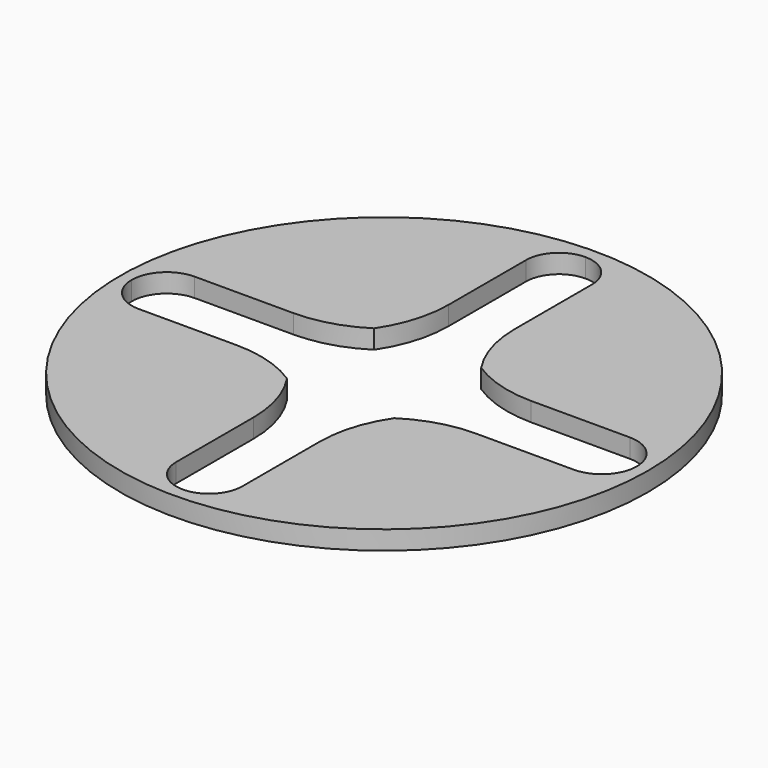
from build123d import *

# Parameters (mm, degrees)
F0_R        = 44.45
F0_R_2      = 12.7
F1_DEPTH    = 3.175
F3_DEPTH    = 25.4
F4_T1_DEPTH = 48.6343800889
F4_T3_DEPTH = 47.4571451006
F4_T5_DEPTH = 47.1924378771


# Not quite as in the source:
# - a fillet or chamfer that OpenCascade refuses, or shapes differently, is made with other operations: its cross-section is extruded or revolved along the edge and cut away or added


with BuildPart() as f1:
    # F0 (on Top) → F1 (new body)
    with BuildSketch(Plane.XY):
        Circle(F0_R)
        Circle(F0_R_2, mode=Mode.SUBTRACT)
    extrude(amount=F1_DEPTH)

    # F2 (on face) → F3 (cut)
    with BuildSketch(Plane.XY.offset(3.175)):
        with BuildLine():
            Line((-42.5250590142, 0), (-12.7, 0))
            ThreePointArc((-12.7, 0), (-12.3276162196, 3.0528475792), (-11.2323026233, 5.9266666667))
            Line((-11.2323026233, 5.9266666667), (-36.6323026233, 5.9266666667))
            ThreePointArc((-36.6323026233, 5.9266666667), (-40.8111169187, 4.1887178728), (-42.5250590142, 0))
        make_face()
        with BuildLine():
            ThreePointArc((-11.2677815117, -5.8589333333), (-12.3367504878, -3.0157233628), (-12.7, 0))
            Line((-12.7, 0), (-42.5250590142, 0))
            ThreePointArc((-42.5250590142, 0), (-40.79976808, -4.1324743979), (-36.6677815117, -5.8589333333))
            Line((-36.6677815117, -5.8589333333), (-11.2677815117, -5.8589333333))
        make_face()
        with BuildLine():
            Line((0, 12.7), (0, 42.3763238149))
            ThreePointArc((0, 42.3763238149), (-3.928862053, 40.7489358679), (-5.55625, 36.8200738149))
            Line((-5.55625, 36.8200738149), (-5.55625, 11.4200738149))
            ThreePointArc((-5.55625, 11.4200738149), (-2.8508825433, 12.3758825433), (0, 12.7))
        make_face()
        with BuildLine():
            ThreePointArc((5.55625, 36.8200738149), (3.928862053, 40.7489358679), (0, 42.3763238149))
            Line((0, 42.3763238149), (0, 12.7))
            ThreePointArc((0, 12.7), (2.8508825433, 12.3758825433), (5.55625, 11.4200738149))
            Line((5.55625, 11.4200738149), (5.55625, 36.8200738149))
        make_face()
        with BuildLine():
            ThreePointArc((5.55625, -11.4200738149), (2.8508825433, -12.3758825433), (0, -12.7))
            Line((0, -12.7), (0, -42.3763238149))
            ThreePointArc((0, -42.3763238149), (3.928862053, -40.7489358679), (5.55625, -36.8200738149))
            Line((5.55625, -36.8200738149), (5.55625, -11.4200738149))
        make_face()
        with BuildLine():
            Line((0, -42.3763238149), (0, -12.7))
            ThreePointArc((0, -12.7), (-2.8508825433, -12.3758825433), (-5.55625, -11.4200738149))
            Line((-5.55625, -11.4200738149), (-5.55625, -36.8200738149))
            ThreePointArc((-5.55625, -36.8200738149), (-3.928862053, -40.7489358679), (0, -42.3763238149))
        make_face()
        with BuildLine():
            ThreePointArc((11.2323026233, 5.9266666667), (12.3276162196, 3.0528475792), (12.7, 0))
            Line((12.7, 0), (42.5250590142, 0))
            ThreePointArc((42.5250590142, 0), (40.8111169187, 4.1887178728), (36.6323026233, 5.9266666667))
            Line((36.6323026233, 5.9266666667), (11.2323026233, 5.9266666667))
        make_face()
        with BuildLine():
            Line((42.5250590142, 0), (12.7, 0))
            ThreePointArc((12.7, 0), (12.3367504878, -3.0157233628), (11.2677815117, -5.8589333333))
            Line((11.2677815117, -5.8589333333), (36.6677815117, -5.8589333333))
            ThreePointArc((36.6677815117, -5.8589333333), (40.79976808, -4.1324743979), (42.5250590142, 0))
        make_face()
    extrude(amount=-F3_DEPTH, mode=Mode.SUBTRACT)

    # F4: fillet of radius 20.32 on 8 edges, made by hand

    # F4_s2 → F4_t1 (cut)
    with BuildSketch(Plane.XY.offset(-22.7296900444)):
        with BuildLine():
            ThreePointArc((-9.9524038462, -7.8892114741), (-6.6867352348, -13.8287677255), (-5.55625, -20.5119498327))
            Line((-5.55625, -20.5119498327), (-5.55625, -11.4200738149))
            ThreePointArc((-5.55625, -11.4200738149), (-7.9527563302, -9.901700195), (-9.9524038462, -7.8892114741))
        make_face()
        with BuildLine():
            ThreePointArc((9.9524038462, 7.8892114741), (6.6867352348, 13.8287677255), (5.55625, 20.5119498327))
            Line((5.55625, 20.5119498327), (5.55625, 11.4200738149))
            ThreePointArc((5.55625, 11.4200738149), (7.9527563302, 9.901700195), (9.9524038462, 7.8892114741))
        make_face()
        with BuildLine():
            ThreePointArc((-5.55625, 20.5119498327), (-6.6867352348, 13.8287677255), (-9.9524038462, 7.8892114741))
            ThreePointArc((-9.9524038462, 7.8892114741), (-7.9527563302, 9.901700195), (-5.55625, 11.4200738149))
            Line((-5.55625, 11.4200738149), (-5.55625, 20.5119498327))
        make_face()
        with BuildLine():
            ThreePointArc((5.55625, -20.5119498327), (6.6867352348, -13.8287677255), (9.9524038462, -7.8892114741))
            ThreePointArc((9.9524038462, -7.8892114741), (7.9527563302, -9.901700195), (5.55625, -11.4200738149))
            Line((5.55625, -11.4200738149), (5.55625, -20.5119498327))
        make_face()
    extrude(amount=F4_T1_DEPTH, mode=Mode.SUBTRACT)

    # F4_s4 → F4_t3 (cut)
    with BuildSketch(Plane.XY.offset(-22.1410725503)):
        with BuildLine():
            ThreePointArc((-20.1242105318, -5.8589333333), (-13.5841452612, -6.9401717761), (-7.7400809738, -10.0688205128))
            ThreePointArc((-7.7400809738, -10.0688205128), (-9.7342435034, -8.1568684811), (-11.2677815117, -5.8589333333))
            Line((-11.2677815117, -5.8589333333), (-20.1242105318, -5.8589333333))
        make_face()
        with BuildLine():
            ThreePointArc((7.7400809738, -10.0688205128), (13.5841452612, -6.9401717761), (20.1242105318, -5.8589333333))
            Line((20.1242105318, -5.8589333333), (11.2677815117, -5.8589333333))
            ThreePointArc((11.2677815117, -5.8589333333), (9.7342435034, -8.1568684811), (7.7400809738, -10.0688205128))
        make_face()
    extrude(amount=F4_T3_DEPTH, mode=Mode.SUBTRACT)

    # F4_s6 → F4_t5 (cut)
    with BuildSketch(Plane.XY.offset(-22.0087189386)):
        with BuildLine():
            ThreePointArc((7.7060731534, 10.0948717949), (13.5281820281, 6.9969020993), (20.0357901988, 5.9266666667))
            Line((20.0357901988, 5.9266666667), (11.2323026233, 5.9266666667))
            ThreePointArc((11.2323026233, 5.9266666667), (9.6958239858, 8.2024994506), (7.7060731534, 10.0948717949))
        make_face()
        with BuildLine():
            ThreePointArc((-7.7060731534, 10.0948717949), (-13.5281820281, 6.9969020993), (-20.0357901988, 5.9266666667))
            Line((-20.0357901988, 5.9266666667), (-11.2323026233, 5.9266666667))
            ThreePointArc((-11.2323026233, 5.9266666667), (-9.6958239858, 8.2024994506), (-7.7060731534, 10.0948717949))
        make_face()
    extrude(amount=F4_T5_DEPTH, mode=Mode.SUBTRACT)


solid = f1.part
